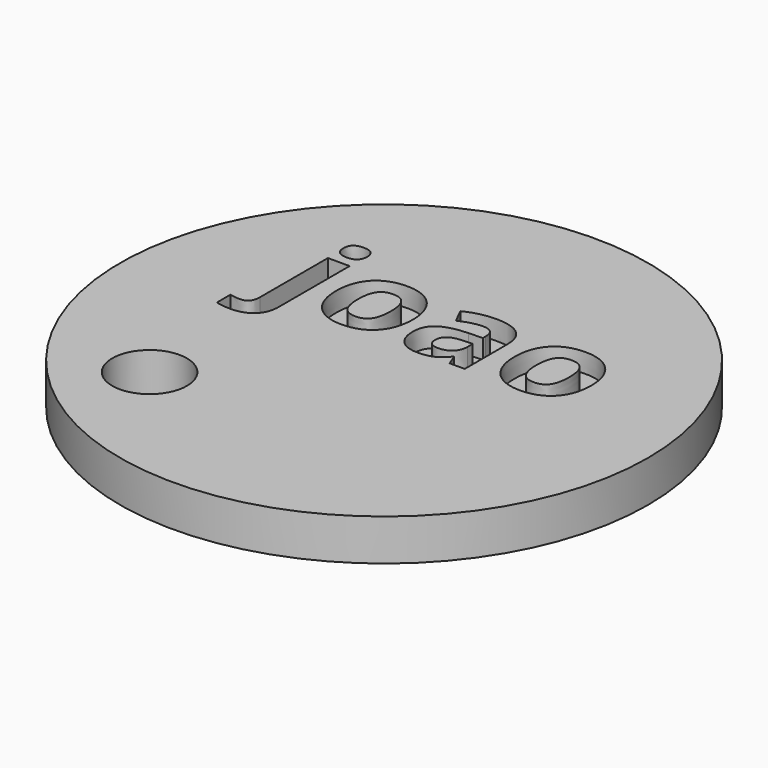
from build123d import *

# Parameters (mm, degrees)
F0_R         = 13.7
F1_DEPTH     = 2.15
F2_R         = 1.9388407712
F2_TEXT_SIZE = 7.5709519377
F3_DEPTH     = 1
F4_DEPTH     = 12.5


# Not quite as in the source:
# - Text() gives the source's letters only with a copy of the font that has no kerning and outlines rounded to 1/6400 em; it was checked with that copy


with BuildPart() as f1:
    # F0 (on Top) → F1 (new body)
    with BuildSketch(Plane.XY):
        Circle(F0_R)
    extrude(amount=F1_DEPTH)

    # F2 (on face) → F3 (cut)
    with BuildSketch(Plane.XY.offset(2.15)):
        with Locations((-6.7828488536, -6.7344135605)):
            Circle(F2_R)
        with Locations((-7.9847676679, 1.4626780758)):
            Text('joao', F2_TEXT_SIZE, font='Open Sans', font_style=FontStyle.BOLD, text_align=(TextAlign.LEFT, TextAlign.BOTTOM))
    extrude(amount=-F3_DEPTH, mode=Mode.SUBTRACT)

    # F2 (on face) → F4 (cut, symmetric)
    with BuildSketch(Plane.XY.offset(2.15)):
        with Locations((-6.7828488536, -6.7344135605)):
            Circle(F2_R)
    extrude(amount=F4_DEPTH, both=True, mode=Mode.SUBTRACT)


solid = f1.part
